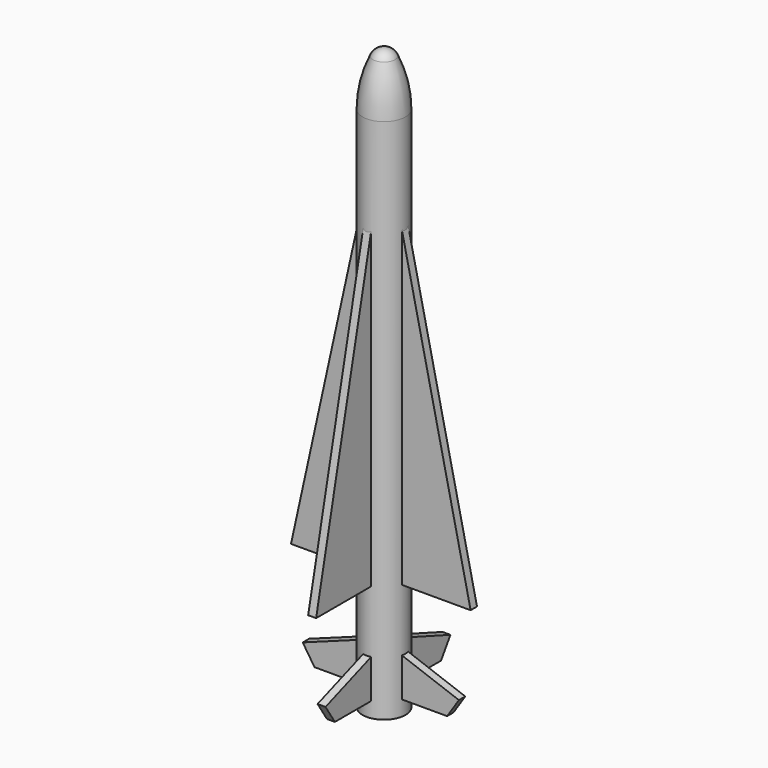
from build123d import *

# Parameters (mm, degrees)
F3_DEPTH     = 0.2
F4_COUNT     = 4
F7_DEPTH     = 10.0694444444
F8_T4_ANGLE  = 140.6790411595
F8_S5_R      = 0.2
F8_T6_DEPTH  = 4
F8_T10_ANGLE = 140.6790411595
F8_S11_R     = 0.2
F8_T12_DEPTH = 4


# Not quite as in the source:
# - a fillet or chamfer that OpenCascade refuses, or shapes differently, is made with other operations: its cross-section is extruded or revolved along the edge and cut away or added


with BuildPart() as f1:
    # F0 (on Front) → F1 (revolve)
    with BuildSketch(Plane.XZ):
        with BuildLine():
            Line((0, 29.1666666667), (0, 0))
            Line((0, 0), (1.0763888889, 0))
            Line((1.0763888889, 0), (1.0763888889, 26.4583333333))
            ThreePointArc((1.0763888889, 26.4583333333), (0.9425798189, 27.6681309336), (0.5476212129, 28.8194444444))
            ThreePointArc((0.5476212129, 28.8194444444), (0.3242114528, 29.0725452046), (0, 29.1666666667))
        make_face()
    revolve(axis=Axis((0, 0, 14.5833333333), (0, 0, 1)))

    # F2 (on Front) → F3 (join, symmetric)
    with BuildSketch(Plane.XZ):
        Polygon((0, 26.351010101), (0, 0.7638888889), (3.3333333333, 0.7638888889), (3.9236111111, 1.6666666667), (1.0763888889, 2.7083333333), (0.4, 2.9557926829), (0.4, 5.8333333333), (4.5138888889, 5.8333333333), align=None)
    extrude(amount=F3_DEPTH, both=True)

    # F4: F1 ×4 about axis
    f4_axis = Axis((0, 0, 0), (0, 0, 1))


with BuildPart() as f1_1:
    add(f1.part)
    for i in range(1, F4_COUNT):
        add(f1.part.rotate(f4_axis, i * 360 / F4_COUNT))

    # F6 (on offset) → F7 (join)
    with BuildSketch(Plane.XY.offset(6)):
        with BuildLine():
            Line((-0.7071923595, -0.424349647), (-0.9025432388, -0.6197005263))
            ThreePointArc((-0.9025432388, -0.6197005263), (-0.9025432388, -0.9025432388), (-0.6197005263, -0.9025432388))
            Line((-0.6197005263, -0.9025432388), (-0.424349647, -0.7071923595))
            Line((-0.424349647, -0.7071923595), (-0.7071923595, -0.424349647))
        make_face()
    extrude(amount=F7_DEPTH)

    # F8: chamfer of 0.25 x 0.4330127019 on 2 edges, made by hand


with BuildPart() as f8_tool2:
    # F8_s3 → F8_t4 (revolve)
    with BuildSketch(Plane(origin=(0, 0, 0), x_dir=(0, 0, 1), z_dir=(0.4279813655, 0.9037875584, 0))):
        with BuildLine():
            Line((16.5174571463, -1.0677286349), (16.0544444444, -1.3350491429))
            Line((16.0544444444, -1.3350491429), (16.0457841904, -1.3350491429))
            ThreePointArc((16.0457841904, -1.3350491429), (16.0607841904, -1.2057190159), (16.0607841904, -1.0763888889))
            Line((16.0607841904, -1.0763888889), (16.0694444444, -1.0677286349))
            ThreePointArc((16.0694444444, -1.0677286349), (16.2934507954, -1.0677286349), (16.5174571463, -1.0590683808))
            Line((16.5174571463, -1.0590683808), (16.5174571463, -1.0677286349))
        make_face()
    revolve(axis=Axis((0, 0, 16.0694444444), (0, 0, 1)), revolution_arc=F8_T4_ANGLE)

    # F8_s5 → F8_t6 (intersect, symmetric)
    with BuildSketch(Plane.XY.offset(16.1)):
        with Locations((-0.7611218825, -0.7611218825)):
            Circle(F8_S5_R)
    extrude(amount=F8_T6_DEPTH, both=True, mode=Mode.INTERSECT)


with BuildPart() as f1_2:
    add(f1_1.part)

    # F8_t1: union F8_tool2
    add(f8_tool2.part)


with BuildPart() as f8_tool8:
    # F8_s9 → F8_t10 (revolve)
    with BuildSketch(Plane(origin=(0, 0, 0), x_dir=(0, 0, 1), z_dir=(0.4279813655, 0.9037875584, 0))):
        with BuildLine():
            Line((5.5519872981, -1.0677286349), (6.015, -1.3350491429))
            Line((6.015, -1.3350491429), (6.023660254, -1.3350491429))
            ThreePointArc((6.023660254, -1.3350491429), (6.008660254, -1.2057190159), (6.008660254, -1.0763888889))
            Line((6.008660254, -1.0763888889), (6, -1.0677286349))
            ThreePointArc((6, -1.0677286349), (5.7759936491, -1.0677286349), (5.5519872981, -1.0590683808))
            Line((5.5519872981, -1.0590683808), (5.5519872981, -1.0677286349))
        make_face()
    revolve(axis=Axis((0, 0, 6), (0, 0, 1)), revolution_arc=F8_T10_ANGLE)

    # F8_s11 → F8_t12 (intersect, symmetric)
    with BuildSketch(Plane.XY.offset(5.9)):
        with Locations((-0.7611218825, -0.7611218825)):
            Circle(F8_S11_R)
    extrude(amount=F8_T12_DEPTH, both=True, mode=Mode.INTERSECT)


with BuildPart() as f1_3:
    add(f1_2.part)

    # F8_t7: union F8_tool8
    add(f8_tool8.part)


solid = f1_3.part
